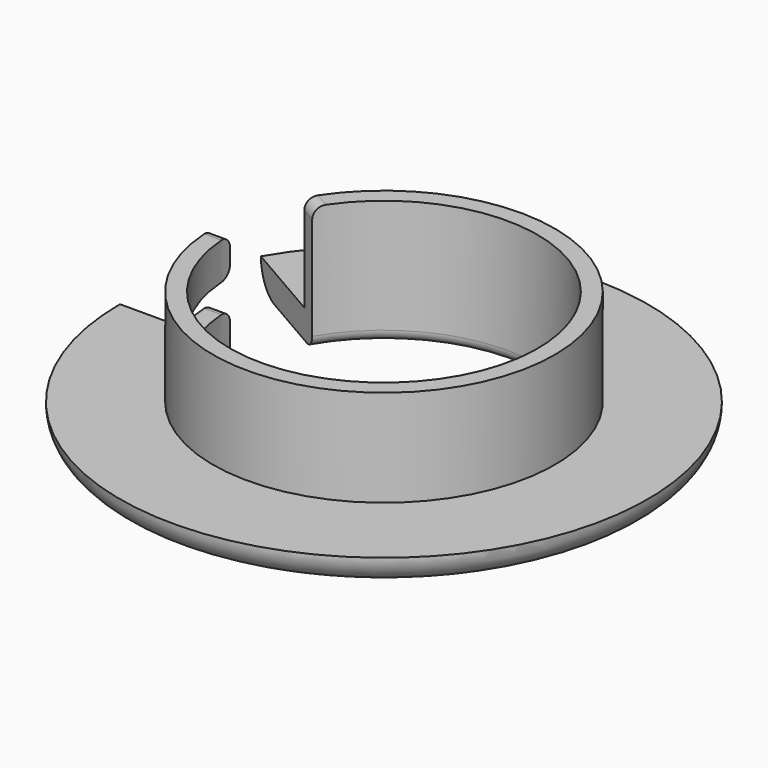
from build123d import *

# Parameters (mm, degrees)
F3_DEPTH      = 17.001
F3_DEPTH_BACK = 25
F5_ANGLE      = -180
F7_DEPTH      = 1.8
F8_DEPTH      = 2.5
F9_R          = 2


with BuildPart() as f1:
    # F0 (on Front) → F1 (revolve)
    with BuildSketch(Plane.XZ):
        with BuildLine():
            Line((-27, 17), (-30, 17))
            Line((-30, 17), (-30, 0))
            Line((-30, 0), (-46.3279513852, 0))
            ThreePointArc((-46.3279513852, 0), (-44.8634852911, -3.5355339059), (-41.3279513852, -5))
            Line((-41.3279513852, -5), (-29, -5))
            ThreePointArc((-29, -5), (-27.5857864376, -4.4142135624), (-27, -3))
            Line((-27, -3), (-27, 17))
        make_face()
    revolve(axis=Axis((0, 0, 7.2955568321), (0, 0, 1)))

    # F2 (on Top) → F3 (cut, two sides)
    with BuildSketch(Plane.XY) as f3_sk:
        Polygon((55.203495074, 0), (0, 0), (55.203495074, -31.8717527412), align=None)
    extrude(amount=F3_DEPTH, mode=Mode.SUBTRACT)
    extrude(f3_sk.sketch, amount=-F3_DEPTH_BACK, mode=Mode.SUBTRACT)


with BuildPart() as f1_1:
    # F5: moved
    add(f1.part.rotate(Axis((0, 0, 17), (0, 0, -1)), F5_ANGLE))

    # F6 (on offset) → F7 (join, symmetric)
    with BuildSketch(Plane.XY.offset(8)):
        with BuildLine():
            ThreePointArc((23.1822198309, -6.2116570825), (22.1731087803, -9.1844023768), (20.7846096908, -12))
            Line((20.7846096908, -12), (24.0563691046, -13.8889511783))
            Line((24.0563691046, -13.8889511783), (26.818160989, -7.1859045795))
            Line((26.818160989, -7.1859045795), (23.1822198309, -6.2116570825))
        make_face()
    extrude(amount=F7_DEPTH, both=True)

    # F6 (on offset) → F8 (cut, symmetric)
    with BuildSketch(Plane.XY.offset(8)):
        Polygon((-34.1305090562, -19.7052585912), (0, 0), (-34.9063649774, 6.3153640367), align=None)
    extrude(amount=F8_DEPTH, both=True, mode=Mode.SUBTRACT)

    # F9
    f9_edges = [f1_1.edges().sort_by_distance(p)[0] for p in [
        (-28.5, 0, 5.5),
        (-28.5, 0, 10.5),
        (-28.5, 0, 17),
        (-24.681724, 14.25, 17),
    ]]
    fillet(f9_edges, radius=F9_R)


solid = f1_1.part
